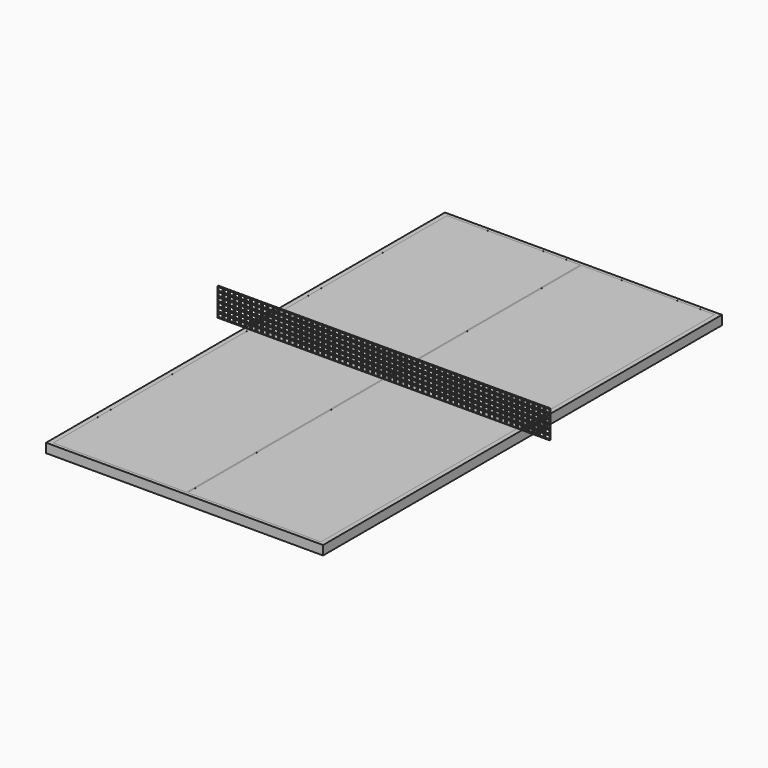
from build123d import *

# Parameters (mm, degrees)
F0_W     = 1524
F0_H     = 2743.2
F1_DEPTH = 25.4
F2_W     = 152.4
F2_H     = 6.35
F2_W_2   = 1524
F3_DEPTH = 152.4
F4_W     = 25.4
F4_H     = 20.32
F5_DEPTH = 1374.776
F7_DEPTH = 0.0254


with BuildPart() as f1:
    # F0 (on Top) → F1 (new body, symmetric)
    with BuildSketch(Plane.XY):
        Rectangle(F0_W, F0_H)
    extrude(amount=F1_DEPTH, both=True)

    # F2 (on face) → F3 (join)
    with BuildSketch(Plane.XY.offset(25.4)):
        with Locations((-838.2, 0)):
            Rectangle(F2_W, F2_H)
        Rectangle(F2_W_2, F2_H)
        with Locations((838.2, 0)):
            Rectangle(F2_W, F2_H)
    extrude(amount=F3_DEPTH)

    # F4 (on face) → F5 (cut, through all)
    with BuildSketch(Plane.XZ.offset(3.175)):
        with Locations((-899.16, 165.1)):
            Rectangle(F4_W, F4_H)
        with Locations((-868.68, 165.1)):
            Rectangle(F4_W, F4_H)
        with Locations((-838.2, 165.1)):
            Rectangle(F4_W, F4_H)
        with Locations((-807.72, 165.1)):
            Rectangle(F4_W, F4_H)
        with Locations((-777.24, 165.1)):
            Rectangle(F4_W, F4_H)
        with Locations((-746.76, 165.1)):
            Rectangle(F4_W, F4_H)
        with Locations((-716.28, 165.1)):
            Rectangle(F4_W, F4_H)
        with Locations((-685.8, 165.1)):
            Rectangle(F4_W, F4_H)
        with Locations((-655.32, 165.1)):
            Rectangle(F4_W, F4_H)
        with Locations((-624.84, 165.1)):
            Rectangle(F4_W, F4_H)
        with Locations((-594.36, 165.1)):
            Rectangle(F4_W, F4_H)
        with Locations((-563.88, 165.1)):
            Rectangle(F4_W, F4_H)
        with Locations((-533.4, 165.1)):
            Rectangle(F4_W, F4_H)
        with Locations((-502.92, 165.1)):
            Rectangle(F4_W, F4_H)
        with Locations((-472.44, 165.1)):
            Rectangle(F4_W, F4_H)
        with Locations((-441.96, 165.1)):
            Rectangle(F4_W, F4_H)
        with Locations((-411.48, 165.1)):
            Rectangle(F4_W, F4_H)
        with Locations((-381, 165.1)):
            Rectangle(F4_W, F4_H)
        with Locations((-350.52, 165.1)):
            Rectangle(F4_W, F4_H)
        with Locations((-320.04, 165.1)):
            Rectangle(F4_W, F4_H)
        with Locations((-289.56, 165.1)):
            Rectangle(F4_W, F4_H)
        with Locations((-259.08, 165.1)):
            Rectangle(F4_W, F4_H)
        with Locations((-228.6, 165.1)):
            Rectangle(F4_W, F4_H)
        with Locations((-198.12, 165.1)):
            Rectangle(F4_W, F4_H)
        with Locations((-167.64, 165.1)):
            Rectangle(F4_W, F4_H)
        with Locations((-137.16, 165.1)):
            Rectangle(F4_W, F4_H)
        with Locations((-106.68, 165.1)):
            Rectangle(F4_W, F4_H)
        with Locations((-76.2, 165.1)):
            Rectangle(F4_W, F4_H)
        with Locations((-45.72, 165.1)):
            Rectangle(F4_W, F4_H)
        with Locations((-15.24, 165.1)):
            Rectangle(F4_W, F4_H)
        with Locations((15.24, 165.1)):
            Rectangle(F4_W, F4_H)
        with Locations((45.72, 165.1)):
            Rectangle(F4_W, F4_H)
        with Locations((76.2, 165.1)):
            Rectangle(F4_W, F4_H)
        with Locations((106.68, 165.1)):
            Rectangle(F4_W, F4_H)
        with Locations((137.16, 165.1)):
            Rectangle(F4_W, F4_H)
        with Locations((167.64, 165.1)):
            Rectangle(F4_W, F4_H)
        with Locations((198.12, 165.1)):
            Rectangle(F4_W, F4_H)
        with Locations((228.6, 165.1)):
            Rectangle(F4_W, F4_H)
        with Locations((259.08, 165.1)):
            Rectangle(F4_W, F4_H)
        with Locations((289.56, 165.1)):
            Rectangle(F4_W, F4_H)
        with Locations((320.04, 165.1)):
            Rectangle(F4_W, F4_H)
        with Locations((350.52, 165.1)):
            Rectangle(F4_W, F4_H)
        with Locations((381, 165.1)):
            Rectangle(F4_W, F4_H)
        with Locations((411.48, 165.1)):
            Rectangle(F4_W, F4_H)
        with Locations((441.96, 165.1)):
            Rectangle(F4_W, F4_H)
        with Locations((472.44, 165.1)):
            Rectangle(F4_W, F4_H)
        with Locations((502.92, 165.1)):
            Rectangle(F4_W, F4_H)
        with Locations((533.4, 165.1)):
            Rectangle(F4_W, F4_H)
        with Locations((563.88, 165.1)):
            Rectangle(F4_W, F4_H)
        with Locations((594.36, 165.1)):
            Rectangle(F4_W, F4_H)
        with Locations((624.84, 165.1)):
            Rectangle(F4_W, F4_H)
        with Locations((655.32, 165.1)):
            Rectangle(F4_W, F4_H)
        with Locations((685.8, 165.1)):
            Rectangle(F4_W, F4_H)
        with Locations((716.28, 165.1)):
            Rectangle(F4_W, F4_H)
        with Locations((746.76, 165.1)):
            Rectangle(F4_W, F4_H)
        with Locations((777.24, 165.1)):
            Rectangle(F4_W, F4_H)
        with Locations((807.72, 165.1)):
            Rectangle(F4_W, F4_H)
        with Locations((838.2, 165.1)):
            Rectangle(F4_W, F4_H)
        with Locations((868.68, 165.1)):
            Rectangle(F4_W, F4_H)
        with Locations((899.16, 165.1)):
            Rectangle(F4_W, F4_H)
        with Locations((899.16, 139.7)):
            Rectangle(F4_W, F4_H)
        with Locations((868.68, 139.7)):
            Rectangle(F4_W, F4_H)
        with Locations((533.4, 139.7)):
            Rectangle(F4_W, F4_H)
        with Locations((411.48, 139.7)):
            Rectangle(F4_W, F4_H)
        with Locations((807.72, 139.7)):
            Rectangle(F4_W, F4_H)
        with Locations((655.32, 139.7)):
            Rectangle(F4_W, F4_H)
        with Locations((777.24, 139.7)):
            Rectangle(F4_W, F4_H)
        with Locations((685.8, 139.7)):
            Rectangle(F4_W, F4_H)
        with Locations((563.88, 139.7)):
            Rectangle(F4_W, F4_H)
        with Locations((441.96, 139.7)):
            Rectangle(F4_W, F4_H)
        with Locations((838.2, 139.7)):
            Rectangle(F4_W, F4_H)
        with Locations((716.28, 139.7)):
            Rectangle(F4_W, F4_H)
        with Locations((594.36, 139.7)):
            Rectangle(F4_W, F4_H)
        with Locations((472.44, 139.7)):
            Rectangle(F4_W, F4_H)
        with Locations((624.84, 139.7)):
            Rectangle(F4_W, F4_H)
        with Locations((502.92, 139.7)):
            Rectangle(F4_W, F4_H)
        with Locations((381, 139.7)):
            Rectangle(F4_W, F4_H)
        with Locations((746.76, 139.7)):
            Rectangle(F4_W, F4_H)
        with Locations((320.04, 139.7)):
            Rectangle(F4_W, F4_H)
        with Locations((198.12, 139.7)):
            Rectangle(F4_W, F4_H)
        with Locations((76.2, 139.7)):
            Rectangle(F4_W, F4_H)
        with Locations((45.72, 139.7)):
            Rectangle(F4_W, F4_H)
        with Locations((167.64, 139.7)):
            Rectangle(F4_W, F4_H)
        with Locations((289.56, 139.7)):
            Rectangle(F4_W, F4_H)
        with Locations((350.52, 139.7)):
            Rectangle(F4_W, F4_H)
        with Locations((228.6, 139.7)):
            Rectangle(F4_W, F4_H)
        with Locations((106.68, 139.7)):
            Rectangle(F4_W, F4_H)
        with Locations((137.16, 139.7)):
            Rectangle(F4_W, F4_H)
        with Locations((15.24, 139.7)):
            Rectangle(F4_W, F4_H)
        with Locations((259.08, 139.7)):
            Rectangle(F4_W, F4_H)
        with Locations((-533.4, 139.7)):
            Rectangle(F4_W, F4_H)
        with Locations((-320.04, 139.7)):
            Rectangle(F4_W, F4_H)
        with Locations((-411.48, 139.7)):
            Rectangle(F4_W, F4_H)
        with Locations((-45.72, 139.7)):
            Rectangle(F4_W, F4_H)
        with Locations((-76.2, 139.7)):
            Rectangle(F4_W, F4_H)
        with Locations((-685.8, 139.7)):
            Rectangle(F4_W, F4_H)
        with Locations((-441.96, 139.7)):
            Rectangle(F4_W, F4_H)
        with Locations((-655.32, 139.7)):
            Rectangle(F4_W, F4_H)
        with Locations((-777.24, 139.7)):
            Rectangle(F4_W, F4_H)
        with Locations((-167.64, 139.7)):
            Rectangle(F4_W, F4_H)
        with Locations((-198.12, 139.7)):
            Rectangle(F4_W, F4_H)
        with Locations((-563.88, 139.7)):
            Rectangle(F4_W, F4_H)
        with Locations((-289.56, 139.7)):
            Rectangle(F4_W, F4_H)
        with Locations((-624.84, 139.7)):
            Rectangle(F4_W, F4_H)
        with Locations((-746.76, 139.7)):
            Rectangle(F4_W, F4_H)
        with Locations((-137.16, 139.7)):
            Rectangle(F4_W, F4_H)
        with Locations((-259.08, 139.7)):
            Rectangle(F4_W, F4_H)
        with Locations((-381, 139.7)):
            Rectangle(F4_W, F4_H)
        with Locations((-502.92, 139.7)):
            Rectangle(F4_W, F4_H)
        with Locations((-15.24, 139.7)):
            Rectangle(F4_W, F4_H)
        with Locations((-350.52, 139.7)):
            Rectangle(F4_W, F4_H)
        with Locations((-472.44, 139.7)):
            Rectangle(F4_W, F4_H)
        with Locations((-594.36, 139.7)):
            Rectangle(F4_W, F4_H)
        with Locations((-716.28, 139.7)):
            Rectangle(F4_W, F4_H)
        with Locations((-106.68, 139.7)):
            Rectangle(F4_W, F4_H)
        with Locations((-228.6, 139.7)):
            Rectangle(F4_W, F4_H)
        with Locations((-807.72, 139.7)):
            Rectangle(F4_W, F4_H)
        with Locations((-899.16, 139.7)):
            Rectangle(F4_W, F4_H)
        with Locations((-868.68, 139.7)):
            Rectangle(F4_W, F4_H)
        with Locations((-838.2, 139.7)):
            Rectangle(F4_W, F4_H)
        with Locations((899.16, 114.3)):
            Rectangle(F4_W, F4_H)
        with Locations((868.68, 114.3)):
            Rectangle(F4_W, F4_H)
        with Locations((533.4, 114.3)):
            Rectangle(F4_W, F4_H)
        with Locations((411.48, 114.3)):
            Rectangle(F4_W, F4_H)
        with Locations((807.72, 114.3)):
            Rectangle(F4_W, F4_H)
        with Locations((655.32, 114.3)):
            Rectangle(F4_W, F4_H)
        with Locations((777.24, 114.3)):
            Rectangle(F4_W, F4_H)
        with Locations((685.8, 114.3)):
            Rectangle(F4_W, F4_H)
        with Locations((563.88, 114.3)):
            Rectangle(F4_W, F4_H)
        with Locations((441.96, 114.3)):
            Rectangle(F4_W, F4_H)
        with Locations((838.2, 114.3)):
            Rectangle(F4_W, F4_H)
        with Locations((716.28, 114.3)):
            Rectangle(F4_W, F4_H)
        with Locations((594.36, 114.3)):
            Rectangle(F4_W, F4_H)
        with Locations((472.44, 114.3)):
            Rectangle(F4_W, F4_H)
        with Locations((624.84, 114.3)):
            Rectangle(F4_W, F4_H)
        with Locations((502.92, 114.3)):
            Rectangle(F4_W, F4_H)
        with Locations((381, 114.3)):
            Rectangle(F4_W, F4_H)
        with Locations((746.76, 114.3)):
            Rectangle(F4_W, F4_H)
        with Locations((320.04, 114.3)):
            Rectangle(F4_W, F4_H)
        with Locations((198.12, 114.3)):
            Rectangle(F4_W, F4_H)
        with Locations((76.2, 114.3)):
            Rectangle(F4_W, F4_H)
        with Locations((45.72, 114.3)):
            Rectangle(F4_W, F4_H)
        with Locations((167.64, 114.3)):
            Rectangle(F4_W, F4_H)
        with Locations((289.56, 114.3)):
            Rectangle(F4_W, F4_H)
        with Locations((350.52, 114.3)):
            Rectangle(F4_W, F4_H)
        with Locations((228.6, 114.3)):
            Rectangle(F4_W, F4_H)
        with Locations((106.68, 114.3)):
            Rectangle(F4_W, F4_H)
        with Locations((137.16, 114.3)):
            Rectangle(F4_W, F4_H)
        with Locations((15.24, 114.3)):
            Rectangle(F4_W, F4_H)
        with Locations((259.08, 114.3)):
            Rectangle(F4_W, F4_H)
        with Locations((-533.4, 114.3)):
            Rectangle(F4_W, F4_H)
        with Locations((-320.04, 114.3)):
            Rectangle(F4_W, F4_H)
        with Locations((-411.48, 114.3)):
            Rectangle(F4_W, F4_H)
        with Locations((-45.72, 114.3)):
            Rectangle(F4_W, F4_H)
        with Locations((-76.2, 114.3)):
            Rectangle(F4_W, F4_H)
        with Locations((-685.8, 114.3)):
            Rectangle(F4_W, F4_H)
        with Locations((-441.96, 114.3)):
            Rectangle(F4_W, F4_H)
        with Locations((-655.32, 114.3)):
            Rectangle(F4_W, F4_H)
        with Locations((-777.24, 114.3)):
            Rectangle(F4_W, F4_H)
        with Locations((-167.64, 114.3)):
            Rectangle(F4_W, F4_H)
        with Locations((-198.12, 114.3)):
            Rectangle(F4_W, F4_H)
        with Locations((-563.88, 114.3)):
            Rectangle(F4_W, F4_H)
        with Locations((-289.56, 114.3)):
            Rectangle(F4_W, F4_H)
        with Locations((-624.84, 114.3)):
            Rectangle(F4_W, F4_H)
        with Locations((-746.76, 114.3)):
            Rectangle(F4_W, F4_H)
        with Locations((-137.16, 114.3)):
            Rectangle(F4_W, F4_H)
        with Locations((-259.08, 114.3)):
            Rectangle(F4_W, F4_H)
        with Locations((-381, 114.3)):
            Rectangle(F4_W, F4_H)
        with Locations((-502.92, 114.3)):
            Rectangle(F4_W, F4_H)
        with Locations((-15.24, 114.3)):
            Rectangle(F4_W, F4_H)
        with Locations((-350.52, 114.3)):
            Rectangle(F4_W, F4_H)
        with Locations((-472.44, 114.3)):
            Rectangle(F4_W, F4_H)
        with Locations((-594.36, 114.3)):
            Rectangle(F4_W, F4_H)
        with Locations((-716.28, 114.3)):
            Rectangle(F4_W, F4_H)
        with Locations((-106.68, 114.3)):
            Rectangle(F4_W, F4_H)
        with Locations((-228.6, 114.3)):
            Rectangle(F4_W, F4_H)
        with Locations((-807.72, 114.3)):
            Rectangle(F4_W, F4_H)
        with Locations((-899.16, 114.3)):
            Rectangle(F4_W, F4_H)
        with Locations((-868.68, 114.3)):
            Rectangle(F4_W, F4_H)
        with Locations((-838.2, 114.3)):
            Rectangle(F4_W, F4_H)
        with Locations((899.16, 88.9)):
            Rectangle(F4_W, F4_H)
        with Locations((868.68, 88.9)):
            Rectangle(F4_W, F4_H)
        with Locations((533.4, 88.9)):
            Rectangle(F4_W, F4_H)
        with Locations((411.48, 88.9)):
            Rectangle(F4_W, F4_H)
        with Locations((807.72, 88.9)):
            Rectangle(F4_W, F4_H)
        with Locations((655.32, 88.9)):
            Rectangle(F4_W, F4_H)
        with Locations((777.24, 88.9)):
            Rectangle(F4_W, F4_H)
        with Locations((685.8, 88.9)):
            Rectangle(F4_W, F4_H)
        with Locations((563.88, 88.9)):
            Rectangle(F4_W, F4_H)
        with Locations((441.96, 88.9)):
            Rectangle(F4_W, F4_H)
        with Locations((838.2, 88.9)):
            Rectangle(F4_W, F4_H)
        with Locations((716.28, 88.9)):
            Rectangle(F4_W, F4_H)
        with Locations((594.36, 88.9)):
            Rectangle(F4_W, F4_H)
        with Locations((472.44, 88.9)):
            Rectangle(F4_W, F4_H)
        with Locations((624.84, 88.9)):
            Rectangle(F4_W, F4_H)
        with Locations((502.92, 88.9)):
            Rectangle(F4_W, F4_H)
        with Locations((381, 88.9)):
            Rectangle(F4_W, F4_H)
        with Locations((746.76, 88.9)):
            Rectangle(F4_W, F4_H)
        with Locations((320.04, 88.9)):
            Rectangle(F4_W, F4_H)
        with Locations((198.12, 88.9)):
            Rectangle(F4_W, F4_H)
        with Locations((76.2, 88.9)):
            Rectangle(F4_W, F4_H)
        with Locations((45.72, 88.9)):
            Rectangle(F4_W, F4_H)
        with Locations((167.64, 88.9)):
            Rectangle(F4_W, F4_H)
        with Locations((289.56, 88.9)):
            Rectangle(F4_W, F4_H)
        with Locations((350.52, 88.9)):
            Rectangle(F4_W, F4_H)
        with Locations((228.6, 88.9)):
            Rectangle(F4_W, F4_H)
        with Locations((106.68, 88.9)):
            Rectangle(F4_W, F4_H)
        with Locations((137.16, 88.9)):
            Rectangle(F4_W, F4_H)
        with Locations((15.24, 88.9)):
            Rectangle(F4_W, F4_H)
        with Locations((259.08, 88.9)):
            Rectangle(F4_W, F4_H)
        with Locations((-533.4, 88.9)):
            Rectangle(F4_W, F4_H)
        with Locations((-320.04, 88.9)):
            Rectangle(F4_W, F4_H)
        with Locations((-411.48, 88.9)):
            Rectangle(F4_W, F4_H)
        with Locations((-45.72, 88.9)):
            Rectangle(F4_W, F4_H)
        with Locations((-76.2, 88.9)):
            Rectangle(F4_W, F4_H)
        with Locations((-685.8, 88.9)):
            Rectangle(F4_W, F4_H)
        with Locations((-441.96, 88.9)):
            Rectangle(F4_W, F4_H)
        with Locations((-655.32, 88.9)):
            Rectangle(F4_W, F4_H)
        with Locations((-777.24, 88.9)):
            Rectangle(F4_W, F4_H)
        with Locations((-167.64, 88.9)):
            Rectangle(F4_W, F4_H)
        with Locations((-198.12, 88.9)):
            Rectangle(F4_W, F4_H)
        with Locations((-563.88, 88.9)):
            Rectangle(F4_W, F4_H)
        with Locations((-289.56, 88.9)):
            Rectangle(F4_W, F4_H)
        with Locations((-624.84, 88.9)):
            Rectangle(F4_W, F4_H)
        with Locations((-746.76, 88.9)):
            Rectangle(F4_W, F4_H)
        with Locations((-137.16, 88.9)):
            Rectangle(F4_W, F4_H)
        with Locations((-259.08, 88.9)):
            Rectangle(F4_W, F4_H)
        with Locations((-381, 88.9)):
            Rectangle(F4_W, F4_H)
        with Locations((-502.92, 88.9)):
            Rectangle(F4_W, F4_H)
        with Locations((-15.24, 88.9)):
            Rectangle(F4_W, F4_H)
        with Locations((-350.52, 88.9)):
            Rectangle(F4_W, F4_H)
        with Locations((-472.44, 88.9)):
            Rectangle(F4_W, F4_H)
        with Locations((-594.36, 88.9)):
            Rectangle(F4_W, F4_H)
        with Locations((-716.28, 88.9)):
            Rectangle(F4_W, F4_H)
        with Locations((-106.68, 88.9)):
            Rectangle(F4_W, F4_H)
        with Locations((-228.6, 88.9)):
            Rectangle(F4_W, F4_H)
        with Locations((-807.72, 88.9)):
            Rectangle(F4_W, F4_H)
        with Locations((-899.16, 88.9)):
            Rectangle(F4_W, F4_H)
        with Locations((-868.68, 88.9)):
            Rectangle(F4_W, F4_H)
        with Locations((-838.2, 88.9)):
            Rectangle(F4_W, F4_H)
        with Locations((899.16, 63.5)):
            Rectangle(F4_W, F4_H)
        with Locations((868.68, 63.5)):
            Rectangle(F4_W, F4_H)
        with Locations((533.4, 63.5)):
            Rectangle(F4_W, F4_H)
        with Locations((411.48, 63.5)):
            Rectangle(F4_W, F4_H)
        with Locations((807.72, 63.5)):
            Rectangle(F4_W, F4_H)
        with Locations((655.32, 63.5)):
            Rectangle(F4_W, F4_H)
        with Locations((777.24, 63.5)):
            Rectangle(F4_W, F4_H)
        with Locations((685.8, 63.5)):
            Rectangle(F4_W, F4_H)
        with Locations((563.88, 63.5)):
            Rectangle(F4_W, F4_H)
        with Locations((441.96, 63.5)):
            Rectangle(F4_W, F4_H)
        with Locations((838.2, 63.5)):
            Rectangle(F4_W, F4_H)
        with Locations((716.28, 63.5)):
            Rectangle(F4_W, F4_H)
        with Locations((594.36, 63.5)):
            Rectangle(F4_W, F4_H)
        with Locations((472.44, 63.5)):
            Rectangle(F4_W, F4_H)
        with Locations((624.84, 63.5)):
            Rectangle(F4_W, F4_H)
        with Locations((502.92, 63.5)):
            Rectangle(F4_W, F4_H)
        with Locations((381, 63.5)):
            Rectangle(F4_W, F4_H)
        with Locations((746.76, 63.5)):
            Rectangle(F4_W, F4_H)
        with Locations((320.04, 63.5)):
            Rectangle(F4_W, F4_H)
        with Locations((198.12, 63.5)):
            Rectangle(F4_W, F4_H)
        with Locations((76.2, 63.5)):
            Rectangle(F4_W, F4_H)
        with Locations((45.72, 63.5)):
            Rectangle(F4_W, F4_H)
        with Locations((167.64, 63.5)):
            Rectangle(F4_W, F4_H)
        with Locations((289.56, 63.5)):
            Rectangle(F4_W, F4_H)
        with Locations((350.52, 63.5)):
            Rectangle(F4_W, F4_H)
        with Locations((228.6, 63.5)):
            Rectangle(F4_W, F4_H)
        with Locations((106.68, 63.5)):
            Rectangle(F4_W, F4_H)
        with Locations((137.16, 63.5)):
            Rectangle(F4_W, F4_H)
        with Locations((15.24, 63.5)):
            Rectangle(F4_W, F4_H)
        with Locations((259.08, 63.5)):
            Rectangle(F4_W, F4_H)
        with Locations((-533.4, 63.5)):
            Rectangle(F4_W, F4_H)
        with Locations((-320.04, 63.5)):
            Rectangle(F4_W, F4_H)
        with Locations((-411.48, 63.5)):
            Rectangle(F4_W, F4_H)
        with Locations((-45.72, 63.5)):
            Rectangle(F4_W, F4_H)
        with Locations((-76.2, 63.5)):
            Rectangle(F4_W, F4_H)
        with Locations((-685.8, 63.5)):
            Rectangle(F4_W, F4_H)
        with Locations((-441.96, 63.5)):
            Rectangle(F4_W, F4_H)
        with Locations((-655.32, 63.5)):
            Rectangle(F4_W, F4_H)
        with Locations((-777.24, 63.5)):
            Rectangle(F4_W, F4_H)
        with Locations((-167.64, 63.5)):
            Rectangle(F4_W, F4_H)
        with Locations((-198.12, 63.5)):
            Rectangle(F4_W, F4_H)
        with Locations((-563.88, 63.5)):
            Rectangle(F4_W, F4_H)
        with Locations((-289.56, 63.5)):
            Rectangle(F4_W, F4_H)
        with Locations((-624.84, 63.5)):
            Rectangle(F4_W, F4_H)
        with Locations((-746.76, 63.5)):
            Rectangle(F4_W, F4_H)
        with Locations((-137.16, 63.5)):
            Rectangle(F4_W, F4_H)
        with Locations((-259.08, 63.5)):
            Rectangle(F4_W, F4_H)
        with Locations((-381, 63.5)):
            Rectangle(F4_W, F4_H)
        with Locations((-502.92, 63.5)):
            Rectangle(F4_W, F4_H)
        with Locations((-15.24, 63.5)):
            Rectangle(F4_W, F4_H)
        with Locations((-350.52, 63.5)):
            Rectangle(F4_W, F4_H)
        with Locations((-472.44, 63.5)):
            Rectangle(F4_W, F4_H)
        with Locations((-594.36, 63.5)):
            Rectangle(F4_W, F4_H)
        with Locations((-716.28, 63.5)):
            Rectangle(F4_W, F4_H)
        with Locations((-106.68, 63.5)):
            Rectangle(F4_W, F4_H)
        with Locations((-228.6, 63.5)):
            Rectangle(F4_W, F4_H)
        with Locations((-807.72, 63.5)):
            Rectangle(F4_W, F4_H)
        with Locations((-899.16, 63.5)):
            Rectangle(F4_W, F4_H)
        with Locations((-868.68, 63.5)):
            Rectangle(F4_W, F4_H)
        with Locations((-838.2, 63.5)):
            Rectangle(F4_W, F4_H)
        with Locations((899.16, 38.1)):
            Rectangle(F4_W, F4_H)
        with Locations((868.68, 38.1)):
            Rectangle(F4_W, F4_H)
        with Locations((533.4, 38.1)):
            Rectangle(F4_W, F4_H)
        with Locations((411.48, 38.1)):
            Rectangle(F4_W, F4_H)
        with Locations((807.72, 38.1)):
            Rectangle(F4_W, F4_H)
        with Locations((655.32, 38.1)):
            Rectangle(F4_W, F4_H)
        with Locations((777.24, 38.1)):
            Rectangle(F4_W, F4_H)
        with Locations((685.8, 38.1)):
            Rectangle(F4_W, F4_H)
        with Locations((563.88, 38.1)):
            Rectangle(F4_W, F4_H)
        with Locations((441.96, 38.1)):
            Rectangle(F4_W, F4_H)
        with Locations((838.2, 38.1)):
            Rectangle(F4_W, F4_H)
        with Locations((716.28, 38.1)):
            Rectangle(F4_W, F4_H)
        with Locations((594.36, 38.1)):
            Rectangle(F4_W, F4_H)
        with Locations((472.44, 38.1)):
            Rectangle(F4_W, F4_H)
        with Locations((624.84, 38.1)):
            Rectangle(F4_W, F4_H)
        with Locations((502.92, 38.1)):
            Rectangle(F4_W, F4_H)
        with Locations((381, 38.1)):
            Rectangle(F4_W, F4_H)
        with Locations((746.76, 38.1)):
            Rectangle(F4_W, F4_H)
        with Locations((320.04, 38.1)):
            Rectangle(F4_W, F4_H)
        with Locations((198.12, 38.1)):
            Rectangle(F4_W, F4_H)
        with Locations((76.2, 38.1)):
            Rectangle(F4_W, F4_H)
        with Locations((45.72, 38.1)):
            Rectangle(F4_W, F4_H)
        with Locations((167.64, 38.1)):
            Rectangle(F4_W, F4_H)
        with Locations((289.56, 38.1)):
            Rectangle(F4_W, F4_H)
        with Locations((350.52, 38.1)):
            Rectangle(F4_W, F4_H)
        with Locations((228.6, 38.1)):
            Rectangle(F4_W, F4_H)
        with Locations((106.68, 38.1)):
            Rectangle(F4_W, F4_H)
        with Locations((137.16, 38.1)):
            Rectangle(F4_W, F4_H)
        with Locations((15.24, 38.1)):
            Rectangle(F4_W, F4_H)
        with Locations((259.08, 38.1)):
            Rectangle(F4_W, F4_H)
        with Locations((-533.4, 38.1)):
            Rectangle(F4_W, F4_H)
        with Locations((-320.04, 38.1)):
            Rectangle(F4_W, F4_H)
        with Locations((-411.48, 38.1)):
            Rectangle(F4_W, F4_H)
        with Locations((-45.72, 38.1)):
            Rectangle(F4_W, F4_H)
        with Locations((-76.2, 38.1)):
            Rectangle(F4_W, F4_H)
        with Locations((-685.8, 38.1)):
            Rectangle(F4_W, F4_H)
        with Locations((-441.96, 38.1)):
            Rectangle(F4_W, F4_H)
        with Locations((-655.32, 38.1)):
            Rectangle(F4_W, F4_H)
        with Locations((-777.24, 38.1)):
            Rectangle(F4_W, F4_H)
        with Locations((-167.64, 38.1)):
            Rectangle(F4_W, F4_H)
        with Locations((-198.12, 38.1)):
            Rectangle(F4_W, F4_H)
        with Locations((-563.88, 38.1)):
            Rectangle(F4_W, F4_H)
        with Locations((-289.56, 38.1)):
            Rectangle(F4_W, F4_H)
        with Locations((-624.84, 38.1)):
            Rectangle(F4_W, F4_H)
        with Locations((-746.76, 38.1)):
            Rectangle(F4_W, F4_H)
        with Locations((-137.16, 38.1)):
            Rectangle(F4_W, F4_H)
        with Locations((-259.08, 38.1)):
            Rectangle(F4_W, F4_H)
        with Locations((-381, 38.1)):
            Rectangle(F4_W, F4_H)
        with Locations((-502.92, 38.1)):
            Rectangle(F4_W, F4_H)
        with Locations((-15.24, 38.1)):
            Rectangle(F4_W, F4_H)
        with Locations((-350.52, 38.1)):
            Rectangle(F4_W, F4_H)
        with Locations((-472.44, 38.1)):
            Rectangle(F4_W, F4_H)
        with Locations((-594.36, 38.1)):
            Rectangle(F4_W, F4_H)
        with Locations((-716.28, 38.1)):
            Rectangle(F4_W, F4_H)
        with Locations((-106.68, 38.1)):
            Rectangle(F4_W, F4_H)
        with Locations((-228.6, 38.1)):
            Rectangle(F4_W, F4_H)
        with Locations((-807.72, 38.1)):
            Rectangle(F4_W, F4_H)
        with Locations((-899.16, 38.1)):
            Rectangle(F4_W, F4_H)
        with Locations((-868.68, 38.1)):
            Rectangle(F4_W, F4_H)
        with Locations((-838.2, 38.1)):
            Rectangle(F4_W, F4_H)
    extrude(amount=-F5_DEPTH, mode=Mode.SUBTRACT)


with BuildPart() as f7:
    # F6 (on face) → F7 (new body)
    with BuildSketch(Plane.XY.offset(25.4)):
        Polygon((-3.1750002625, 1353.820151062), (-3.1750002625, 0), (3.1749997375, 0), (3.1749997375, 1353.820151062), (736.6, 1353.820151062), (736.6, -3.175), (762, -3.175), (762, 1353.820151062), (762, 1371.600151062), (736.6, 1371.600151062), (3.1749997375, 1371.600151062), (-3.1750002625, 1371.600151062), (-736.6, 1371.600151062), (-762, 1371.600151062), (-762, 1353.820151062), (-762, -3.175), (-736.6, -3.175), (-736.6, 1353.820151062), align=None)
        Polygon((3.1749997381, -3.175), (-3.1750002619, -3.175), (-3.1750000034, -1353.82), (-736.6, -1353.82), (-736.6, -3.175), (-762, -3.175), (-762, -1353.82), (-762, -1371.6), (-736.6, -1371.6), (736.6, -1371.6), (762, -1371.6), (762, -1353.82), (762, -3.175), (736.6, -3.175), (736.6, -1353.82), (3.1749999966, -1353.82), align=None)
    extrude(amount=F7_DEPTH)


solid = Compound([f1.part, f7.part])
